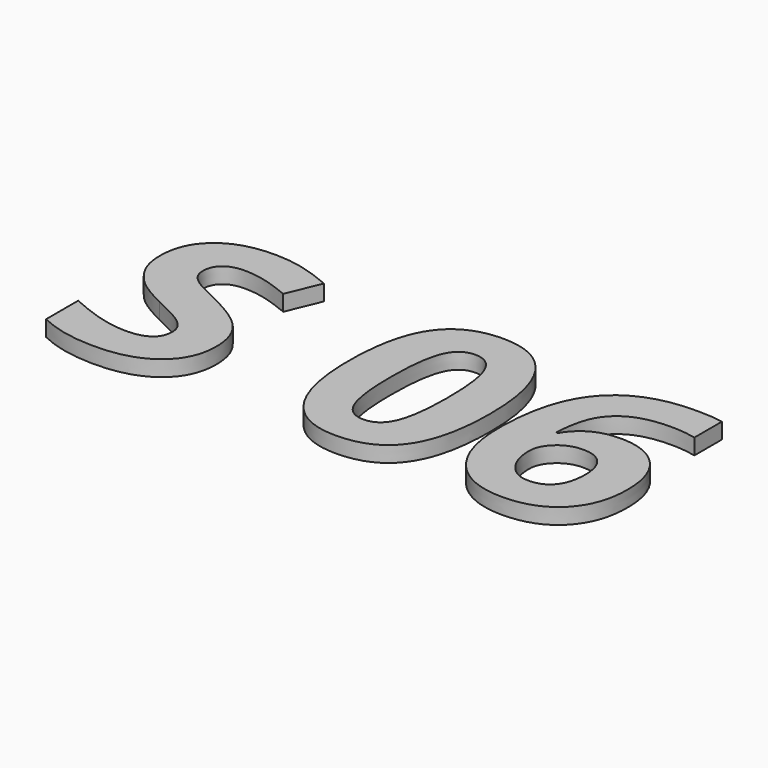
from build123d import *

# Parameters (mm, degrees)
F0_TEXT_SIZE = 18.0555555556
F1_DEPTH     = 1


# Not quite as in the source:
# - Text() gives the source's letters only with a copy of the font that has no kerning and outlines rounded to 1/6400 em; it was checked with that copy


with BuildPart() as f1:
    # F0 (on Top) → F1 (new body)
    with BuildSketch(Plane.XY):
        with Locations((-17.9229600694, -6.5)):
            Text('S 06', F0_TEXT_SIZE, font='Open Sans', font_style=FontStyle.BOLD, text_align=(TextAlign.LEFT, TextAlign.BOTTOM))
    extrude(amount=F1_DEPTH)


solid = f1.part
